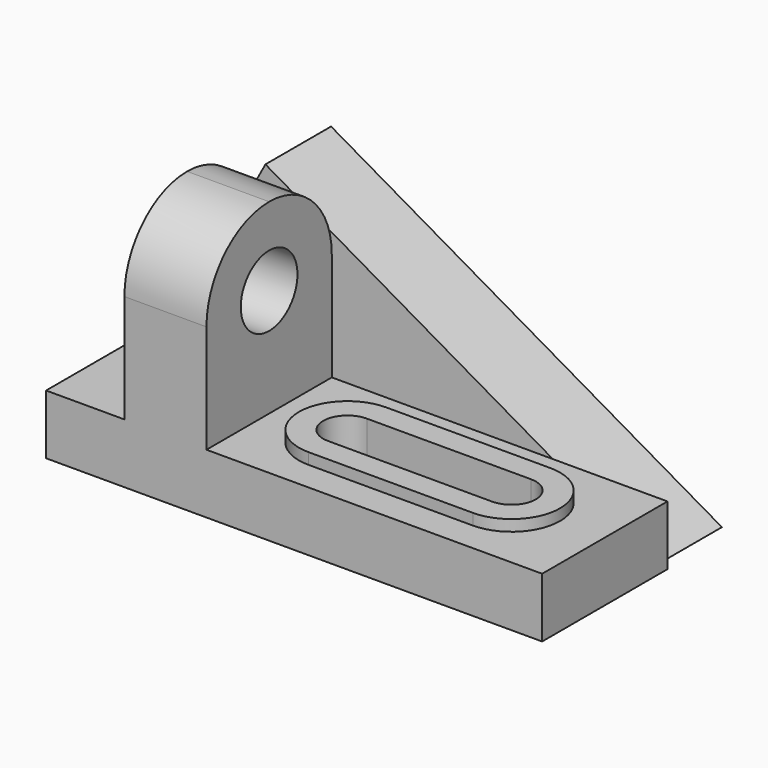
from build123d import *

# Parameters (mm, degrees)
F1_DEPTH  = 42
F3_DEPTH  = 112.001
F4_R      = 9.5
F5_DEPTH  = 112.001
F7_DEPTH  = 3
F9_DEPTH  = 22
F11_DEPTH = 25


with BuildPart() as f1:
    # F0 (on Front) → F1 (new body)
    with BuildSketch(Plane.XZ):
        Polygon((0, 16), (0, 0), (133, 0), (133, 16), (43, 16), (43, 66), (21, 66), (21, 16), align=None)
    extrude(amount=F1_DEPTH)

    # F2 (on face) → F3 (cut, through all)
    with BuildSketch(Plane(origin=(21, 0, 0), x_dir=(0, -1, 0), z_dir=(-1, 0, 0))):
        with BuildLine():
            Line((0, 66), (0, 45))
            ThreePointArc((0, 45), (6.1507575951, 59.8492424049), (21, 66))
            Line((21, 66), (0, 66))
        make_face()
        with BuildLine():
            Line((42, 66), (21, 66))
            ThreePointArc((21, 66), (35.8492424049, 59.8492424049), (42, 45))
            Line((42, 45), (42, 66))
        make_face()
    extrude(amount=-F3_DEPTH, mode=Mode.SUBTRACT)

    # F4 (on face) → F5 (cut, through all)
    with BuildSketch(Plane(origin=(21, 0, 0), x_dir=(0, -1, 0), z_dir=(-1, 0, 0))):
        with Locations((21, 45)):
            Circle(F4_R)
    extrude(amount=-F5_DEPTH, mode=Mode.SUBTRACT)

    # F6 (on face) → F7 (join)
    with BuildSketch(Plane.XY.offset(16)):
        with BuildLine():
            Line((108, -8), (64, -8))
            ThreePointArc((64, -8), (51, -21), (64, -34))
            Line((64, -34), (108, -34))
            ThreePointArc((108, -34), (121, -21), (108, -8))
        make_face()
    extrude(amount=F7_DEPTH)

    # F8 (on Front) → F9 (join)
    with BuildSketch(Plane.XZ):
        with BuildLine():
            ThreePointArc((25.2109261421, 60.5), (13.122975019, 31.3171044574), (9, 0))
            Line((9, 0), (130, 0))
            Line((130, 0), (25.2109261421, 60.5))
        make_face()
    extrude(amount=-F9_DEPTH)

    # F10 (on face) → F11 (cut)
    with BuildSketch(Plane.XY.offset(19)):
        with BuildLine():
            Line((108, -14.5), (64, -14.5))
            ThreePointArc((64, -14.5), (57.5, -21), (64, -27.5))
            Line((64, -27.5), (108, -27.5))
            ThreePointArc((108, -27.5), (114.5, -21), (108, -14.5))
        make_face()
    extrude(amount=-F11_DEPTH, mode=Mode.SUBTRACT)


solid = f1.part
